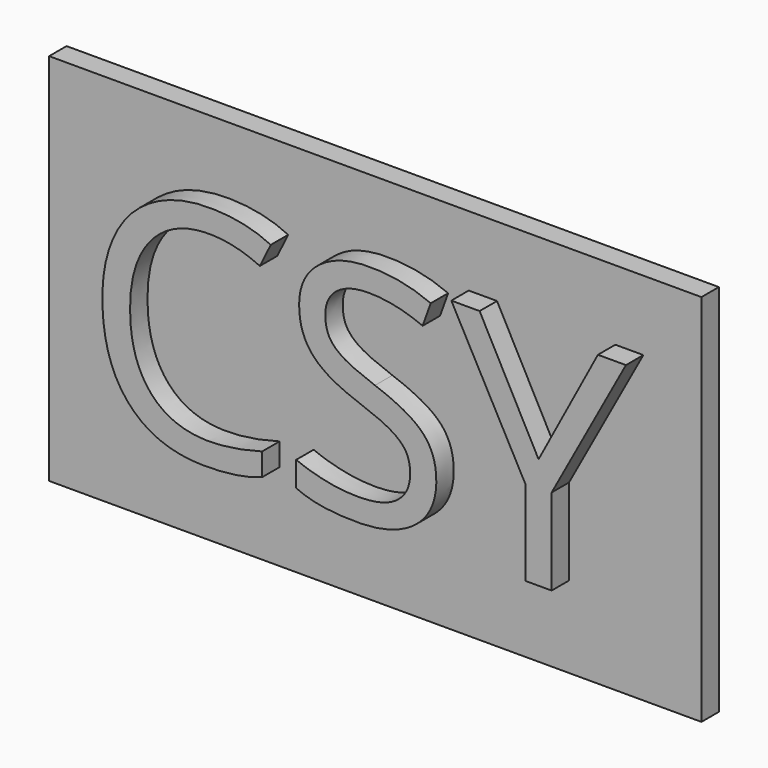
from build123d import *

# Parameters (mm, degrees)
F0_W         = 76.0463699698
F0_H         = 43.5999184847
F1_DEPTH     = 2.54
F2_TEXT_SIZE = 36.3588708246
F3_DEPTH     = 2.54


# Not quite as in the source:
# - Text() gives the source's letters only with a copy of the font that has no kerning and outlines rounded to 1/6400 em; it was checked with that copy


with BuildPart() as f1:
    # F0 (on Front) → F1 (new body)
    with BuildSketch(Plane.XZ):
        with Locations((38.0231849849, 21.7999592423)):
            Rectangle(F0_W, F0_H)
    extrude(amount=F1_DEPTH)

    # F2 (on face) → F3 (join)
    with BuildSketch(Plane.XZ.offset(2.54)):
        with Locations((6.0179363936, 9.4942739233)):
            Text('CSY', F2_TEXT_SIZE, font='Open Sans', text_align=(TextAlign.LEFT, TextAlign.BOTTOM))
    extrude(amount=F3_DEPTH)


solid = f1.part
